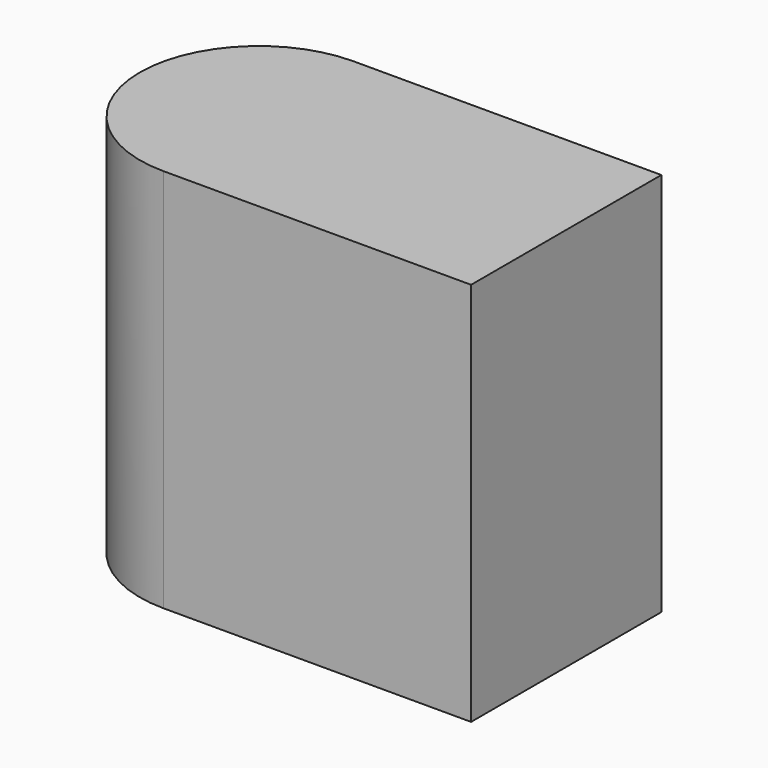
from build123d import *

# Parameters (mm, degrees)
F0_W     = 119.8488399386
F0_H     = 92.6931612194
F1_DEPTH = 150


with BuildPart() as f1:
    # F0 (on Top) → F1 (new body)
    with BuildSketch(Plane.XY):
        with Locations((13.3079923689, 4.1211973876)):
            Rectangle(F0_W, F0_H)
        with BuildLine():
            Line((-46.6164276004, -42.2253832221), (-46.6164276004, 50.4677779973))
            ThreePointArc((-46.6164276004, 50.4677779973), (-92.9630082101, 4.1211973876), (-46.6164276004, -42.2253832221))
        make_face()
    extrude(amount=F1_DEPTH)


solid = f1.part
